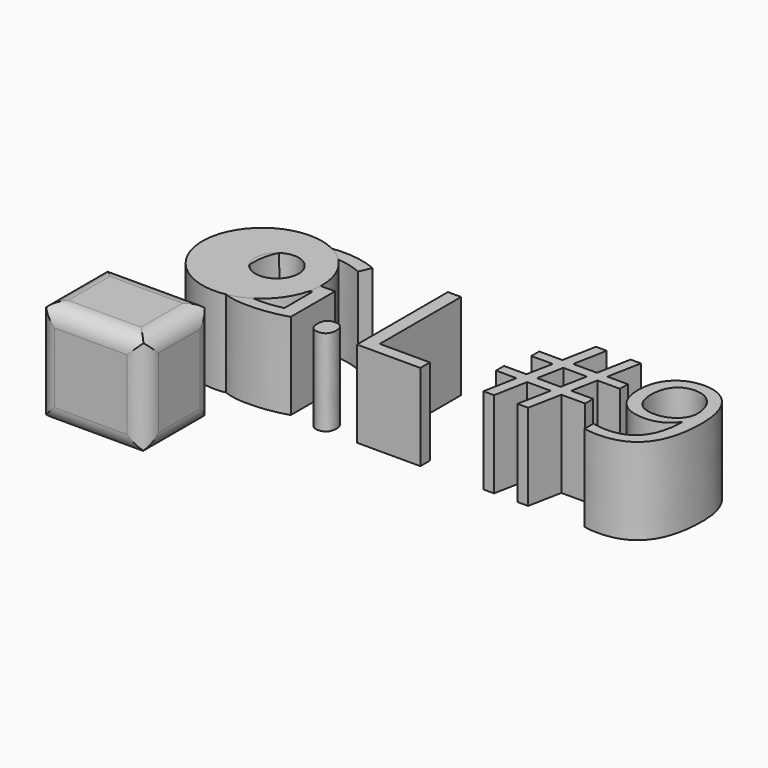
from build123d import *

# Parameters (mm, degrees)
F0_TEXT_SIZE = 46.7477702639
F1_DEPTH     = 25.4
F3_R         = 17.5741578745
F4_DEPTH     = 25.4
F2_W         = 31.5339304507
F2_H         = 30.7504790835
F5_DEPTH     = 25.4
F6_R         = 5.08
F7_R         = 6.378177503
F8_DEPTH     = 25.4
F11_R        = 5.08
F12_T1_DEPTH = 45.9904790835
F13_T1_DEPTH = 45.9904790835
F14_T1_DEPTH = 45.9904790835


# Not quite as in the source:
# - a fillet or chamfer that OpenCascade refuses, or shapes differently, is made with other operations: its cross-section is extruded or revolved along the edge and cut away or added
# - Text() gives the source's letters only with a copy of the font that has no kerning and outlines rounded to 1/6400 em; it was checked with that copy


with BuildPart() as f1:
    # F0 (on Top) → F1 (new body)
    with BuildSketch(Plane.XY):
        with Locations((-54.1957207024, 23.2471134514)):
            Text('G.L #9', F0_TEXT_SIZE, font='Open Sans', text_align=(TextAlign.LEFT, TextAlign.BOTTOM))
    extrude(amount=F1_DEPTH)


with BuildPart() as f4:
    # F3 (on Top) → F4 (new body)
    with BuildSketch(Plane.XY):
        with Locations((-45.3532636166, 41.2172712386)):
            Circle(F3_R)
    extrude(amount=F4_DEPTH)

    # F7 (on face) → F8 (cut)
    with BuildSketch(Plane.XY.offset(25.4)):
        with Locations((-41.9303737581, 42.35823825)):
            Circle(F7_R)
    extrude(amount=-F8_DEPTH, mode=Mode.SUBTRACT)


with BuildPart() as f5:
    # F2 (on Front) → F5 (new body)
    with BuildSketch(Plane.XZ):
        with Locations((-42.4043219537, 22.9159614537)):
            Rectangle(F2_W, F2_H)
    extrude(amount=F5_DEPTH)

    # F6
    f6_edges = [f5.edges().sort_by_distance(p)[0] for p in [
        (-58.171287, -12.7, 7.540722),
        (-26.637357, -12.7, 7.540722),
        (-42.404322, 0, 7.540722),
        (-42.404322, -25.4, 7.540722),
    ]]
    fillet(f6_edges, radius=F6_R)

    # F11
    f11_edges = [f5.edges().sort_by_distance(p)[0] for p in [
        (-26.637357, -12.7, 38.291201),
        (-58.171287, -12.7, 38.291201),
        (-42.404322, 0, 38.291201),
        (-42.404322, -25.4, 38.291201),
    ]]
    fillet(f11_edges, radius=F11_R)

    # F12: fillet of radius 5.08 on 4 edges, made by hand

    # F12_s2 → F12_t1 (cut)
    with BuildSketch(Plane.XY.offset(-0.0792780881)):
        with BuildLine():
            ThreePointArc((-58.171287179, -5.08), (-56.6833896274, -1.4878975516), (-53.091287179, 0))
            Line((-53.091287179, 0), (-58.171287179, 0))
            Line((-58.171287179, 0), (-58.171287179, -5.08))
        make_face()
        with BuildLine():
            ThreePointArc((-58.171287179, -20.32), (-56.6833896274, -23.9121024484), (-53.091287179, -25.4))
            Line((-53.091287179, -25.4), (-58.171287179, -25.4))
            Line((-58.171287179, -25.4), (-58.171287179, -20.32))
        make_face()
    extrude(amount=F12_T1_DEPTH, mode=Mode.SUBTRACT)

    # F13: fillet of radius 5.08 on 4 edges, made by hand

    # F13_s2 → F13_t1 (cut)
    with BuildSketch(Plane.XY.offset(-0.0792780881)):
        with BuildLine():
            ThreePointArc((-31.7173567283, -25.4), (-28.1252542799, -23.9121024484), (-26.6373567283, -20.32))
            Line((-26.6373567283, -20.32), (-26.6373567283, -25.4))
            Line((-26.6373567283, -25.4), (-31.7173567283, -25.4))
        make_face()
    extrude(amount=F13_T1_DEPTH, mode=Mode.SUBTRACT)

    # F14: fillet of radius 5.08 on 4 edges, made by hand

    # F14_s2 → F14_t1 (cut)
    with BuildSketch(Plane.XY.offset(-0.0792780881)):
        with BuildLine():
            ThreePointArc((-31.7173567283, 0), (-28.1252542799, -1.4878975516), (-26.6373567283, -5.08))
            Line((-26.6373567283, -5.08), (-26.6373567283, 0))
            Line((-26.6373567283, 0), (-31.7173567283, 0))
        make_face()
    extrude(amount=F14_T1_DEPTH, mode=Mode.SUBTRACT)


solid = Compound([f1.part, f4.part, f5.part])
